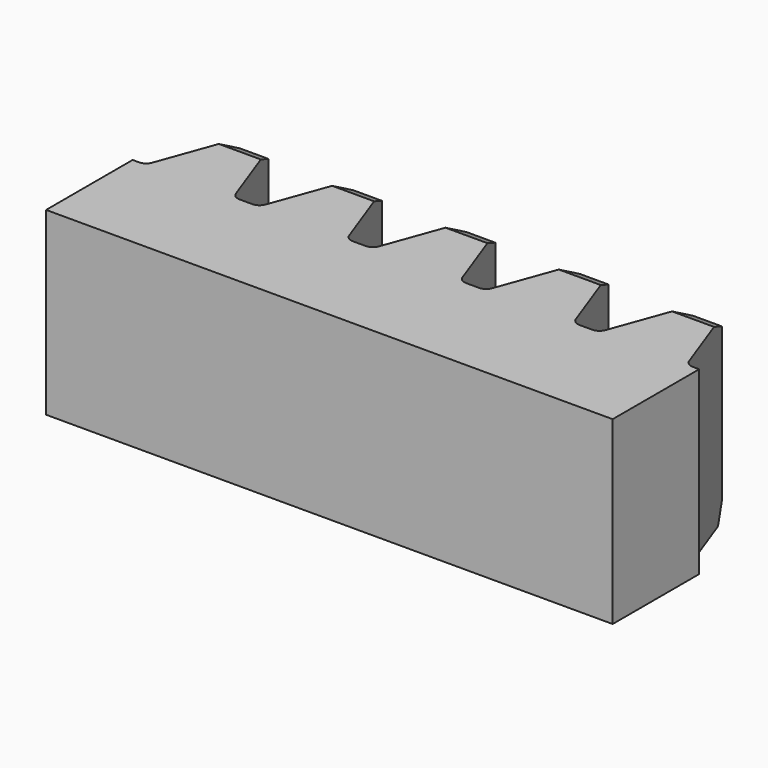
from build123d import *

# Parameters (mm, degrees)
F1_DEPTH     = 5
F2_C1_SIZE2  = 0.25
F2_C1_SIZE   = 0.5
F2_C2_SIZE2  = 0.5
F2_C2_SIZE   = 0.25
F2_C3_SIZE2  = 0.5
F2_C3_SIZE   = 0.25
F2_C4_SIZE2  = 0.5
F2_C4_SIZE   = 0.25
F2_C5_SIZE2  = 0.25
F2_C5_SIZE   = 0.5
F2_C6_SIZE2  = 0.5
F2_C6_SIZE   = 0.25
F2_C7_SIZE2  = 0.5
F2_C7_SIZE   = 0.25
F2_C8_SIZE2  = 0.5
F2_C8_SIZE   = 0.25
F2_C9_SIZE2  = 0.5
F2_C9_SIZE   = 0.25
F2_C10_SIZE2 = 0.5
F2_C10_SIZE  = 0.25


with BuildPart() as f1:
    # F0 (on Top) → F1 (new body)
    with BuildSketch(Plane.XY):
        with BuildLine():
            Line((1.236000562, -12.0934582279), (0.4769388315, -14.1789632613))
            ThreePointArc((0.4769388315, -14.1789632613), (0.3854097856, -14.2982462382), (0.2420156754, -14.3434582279))
            Line((0.2420156754, -14.3434582279), (0.065349562, -14.3434582279))
            Line((0.065349562, -14.3434582279), (0.065349562, -17.3434582279))
            Line((0.065349562, -17.3434582279), (15.773299562, -17.3434582279))
            Line((15.773299562, -17.3434582279), (15.773299562, -14.3434582279))
            Line((15.773299562, -14.3434582279), (15.5966334485, -14.3434582279))
            ThreePointArc((15.5966334485, -14.3434582279), (15.4532393383, -14.2982462382), (15.3617102924, -14.1789632613))
            Line((15.3617102924, -14.1789632613), (14.602648562, -12.0934582279))
            Line((14.602648562, -12.0934582279), (13.802360562, -12.0934582279))
            Line((13.802360562, -12.0934582279), (13.0432988315, -14.1789632613))
            ThreePointArc((13.0432988315, -14.1789632613), (12.9517697856, -14.2982462382), (12.8083756754, -14.3434582279))
            Line((12.8083756754, -14.3434582279), (12.4550434485, -14.3434582279))
            ThreePointArc((12.4550434485, -14.3434582279), (12.3116493383, -14.2982462382), (12.2201202924, -14.1789632613))
            Line((12.2201202924, -14.1789632613), (11.461058562, -12.0934582279))
            Line((11.461058562, -12.0934582279), (10.660770562, -12.0934582279))
            Line((10.660770562, -12.0934582279), (9.9017088315, -14.1789632613))
            ThreePointArc((9.9017088315, -14.1789632613), (9.8101797856, -14.2982462382), (9.6667856754, -14.3434582279))
            Line((9.6667856754, -14.3434582279), (9.3134534485, -14.3434582279))
            ThreePointArc((9.3134534485, -14.3434582279), (9.1700593383, -14.2982462382), (9.0785302924, -14.1789632613))
            Line((9.0785302924, -14.1789632613), (8.319468562, -12.0934582279))
            Line((8.319468562, -12.0934582279), (7.519180562, -12.0934582279))
            Line((7.519180562, -12.0934582279), (6.7601188315, -14.1789632613))
            ThreePointArc((6.7601188315, -14.1789632613), (6.6685897856, -14.2982462382), (6.5251956754, -14.3434582279))
            Line((6.5251956754, -14.3434582279), (6.1718634485, -14.3434582279))
            ThreePointArc((6.1718634485, -14.3434582279), (6.0284693383, -14.2982462382), (5.9369402924, -14.1789632613))
            Line((5.9369402924, -14.1789632613), (5.177878562, -12.0934582279))
            Line((5.177878562, -12.0934582279), (4.377590562, -12.0934582279))
            Line((4.377590562, -12.0934582279), (3.6185288315, -14.1789632613))
            ThreePointArc((3.6185288315, -14.1789632613), (3.5269997856, -14.2982462382), (3.3836056754, -14.3434582279))
            Line((3.3836056754, -14.3434582279), (3.0302734485, -14.3434582279))
            ThreePointArc((3.0302734485, -14.3434582279), (2.8868793383, -14.2982462382), (2.7953502924, -14.1789632613))
            Line((2.7953502924, -14.1789632613), (2.036288562, -12.0934582279))
            Line((2.036288562, -12.0934582279), (1.236000562, -12.0934582279))
        make_face()
    extrude(amount=F1_DEPTH)

    # F2: chamfer of 0.25 x 0.5 on 10 edges, made by hand

    # F2_c1
    f2_c1_edges = [f1.edges().sort_by_distance(p)[0] for p in [
        (7.919324562, -12.0934582279, 0),
    ]]
    f2_c1_side = f1.faces().sort_by_distance((7.919324562, -12.0934582279, 0.005))[0]
    chamfer(f2_c1_edges, length=F2_C1_SIZE, length2=F2_C1_SIZE2, reference=f2_c1_side)

    # F2_c2
    f2_c2_edges = [f1.edges().sort_by_distance(p)[0] for p in [
        (7.919324562, -12.0934582279, 5),
    ]]
    f2_c2_side = f1.faces().sort_by_distance((7.919324562, -12.0934582279, 4.995))[0]
    chamfer(f2_c2_edges, length=F2_C2_SIZE, length2=F2_C2_SIZE2, reference=f2_c2_side)

    # F2_c3
    f2_c3_edges = [f1.edges().sort_by_distance(p)[0] for p in [
        (4.777734562, -12.0934582279, 0),
    ]]
    f2_c3_side = f1.faces().sort_by_distance((4.777734562, -12.0984582279, 0))[0]
    chamfer(f2_c3_edges, length=F2_C3_SIZE, length2=F2_C3_SIZE2, reference=f2_c3_side)

    # F2_c4
    f2_c4_edges = [f1.edges().sort_by_distance(p)[0] for p in [
        (4.777734562, -12.0934582279, 5),
    ]]
    f2_c4_side = f1.faces().sort_by_distance((4.777734562, -12.0934582279, 4.995))[0]
    chamfer(f2_c4_edges, length=F2_C4_SIZE, length2=F2_C4_SIZE2, reference=f2_c4_side)

    # F2_c5
    f2_c5_edges = [f1.edges().sort_by_distance(p)[0] for p in [
        (1.636144562, -12.0934582279, 0),
    ]]
    f2_c5_side = f1.faces().sort_by_distance((1.636144562, -12.0984582279, 0))[0]
    chamfer(f2_c5_edges, length=F2_C5_SIZE, length2=F2_C5_SIZE2, reference=f2_c5_side)

    # F2_c6
    f2_c6_edges = [f1.edges().sort_by_distance(p)[0] for p in [
        (1.636144562, -12.0934582279, 5),
    ]]
    f2_c6_side = f1.faces().sort_by_distance((1.636144562, -12.0934582279, 4.995))[0]
    chamfer(f2_c6_edges, length=F2_C6_SIZE, length2=F2_C6_SIZE2, reference=f2_c6_side)

    # F2_c7
    f2_c7_edges = [f1.edges().sort_by_distance(p)[0] for p in [
        (14.202504562, -12.0934582279, 0),
    ]]
    f2_c7_side = f1.faces().sort_by_distance((14.202504562, -12.0984582279, 0))[0]
    chamfer(f2_c7_edges, length=F2_C7_SIZE, length2=F2_C7_SIZE2, reference=f2_c7_side)

    # F2_c8
    f2_c8_edges = [f1.edges().sort_by_distance(p)[0] for p in [
        (14.202504562, -12.0934582279, 5),
    ]]
    f2_c8_side = f1.faces().sort_by_distance((14.202504562, -12.0934582279, 4.995))[0]
    chamfer(f2_c8_edges, length=F2_C8_SIZE, length2=F2_C8_SIZE2, reference=f2_c8_side)

    # F2_c9
    f2_c9_edges = [f1.edges().sort_by_distance(p)[0] for p in [
        (11.060914562, -12.0934582279, 0),
    ]]
    f2_c9_side = f1.faces().sort_by_distance((11.060914562, -12.0984582279, 0))[0]
    chamfer(f2_c9_edges, length=F2_C9_SIZE, length2=F2_C9_SIZE2, reference=f2_c9_side)

    # F2_c10
    f2_c10_edges = [f1.edges().sort_by_distance(p)[0] for p in [
        (11.060914562, -12.0934582279, 5),
    ]]
    f2_c10_side = f1.faces().sort_by_distance((11.060914562, -12.0934582279, 4.995))[0]
    chamfer(f2_c10_edges, length=F2_C10_SIZE, length2=F2_C10_SIZE2, reference=f2_c10_side)


solid = f1.part
